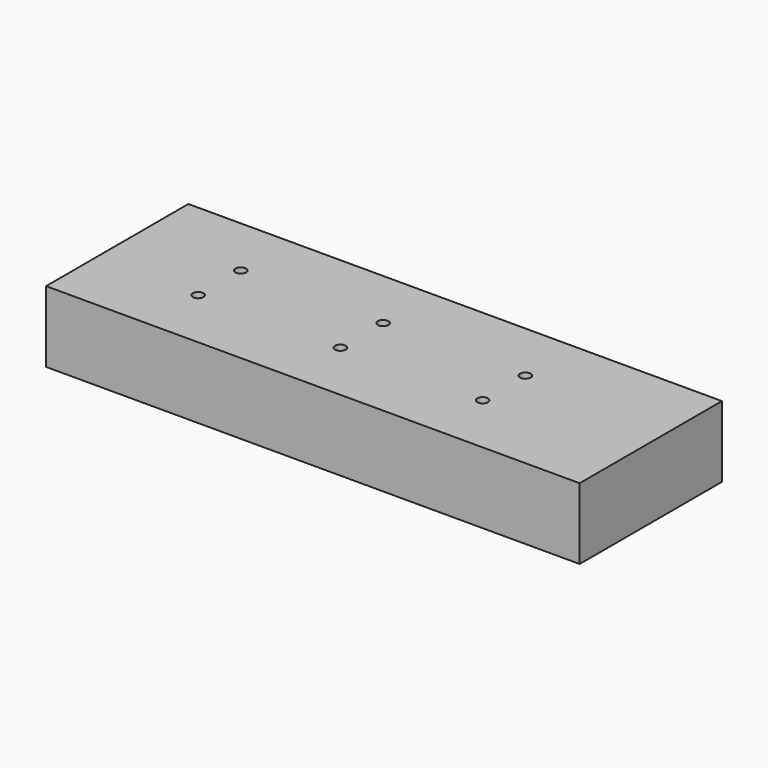
from build123d import *

# Parameters (mm, degrees)
F0_W     = 76.2
F0_H     = 25.4
F1_DEPTH = 10.16
F2_R     = 6.35
F3_DEPTH = 3.81


# Not quite as in the source:
# - a pattern or mirror of a feature is missing from the dataset's text; its kind, count and spacing are read off the source's solid


with BuildPart() as f1:
    # F0 (on Top) → F1 (new body)
    with BuildSketch(Plane.XY):
        Rectangle(F0_W, F0_H)
    extrude(amount=F1_DEPTH)

    # F2 (on face) → F3 (cut)
    with BuildSketch(Plane(origin=(0, 0, 0), x_dir=(1, 0, 0), z_dir=(0, 0, -1))):
        with Locations((-23.495, 0)):
            Circle(F2_R)
        with Locations((-3.175, 0)):
            Circle(F2_R)
        with Locations((17.145, 0)):
            Circle(F2_R)
    extrude(amount=-F3_DEPTH, mode=Mode.SUBTRACT)

    # F5 (on offset) → F6 (revolve, cut)
    with BuildSketch(Plane.XZ.offset(3.81)):
        Polygon((-26.035, 3.81), (-23.495, 3.81), (-23.495, 10.4205608368), (-24.257, 10.4205608368), (-24.257, 4.4571390765), align=None)
    f6 = revolve(axis=Axis((-23.495, -3.81, 7.1152804184), (0, 0, -1)), mode=Mode.SUBTRACT)

    # F6_copies: F6 across plane
    add(f6.mirror(Plane.ZX), mode=Mode.SUBTRACT)

    # F7 (on offset) → F8 (revolve, cut)
    with BuildSketch(Plane.XZ.offset(3.81)):
        Polygon((-5.715, 3.81), (-3.175, 3.81), (-3.175, 10.4205607442), (-3.937, 10.4205607442), (-3.937, 4.4571389839), align=None)
    f8 = revolve(axis=Axis((-3.175, -3.81, 10.0472030926), (0, 0, 1)), mode=Mode.SUBTRACT)

    # F8_copies: F8 across plane
    add(f8.mirror(Plane.ZX), mode=Mode.SUBTRACT)

    # F9 (on offset) → F10 (revolve, cut)
    with BuildSketch(Plane.XZ.offset(3.81)):
        Polygon((14.605, 3.81), (17.145, 3.81), (17.145, 10.4205608368), (16.383, 10.4205608368), (16.383, 4.4571390765), align=None)
    f10 = revolve(axis=Axis((17.145, -3.81, 8.0366932552), (0, 0, 1)), mode=Mode.SUBTRACT)

    # F10_copies: F10 across plane
    add(f10.mirror(Plane.ZX), mode=Mode.SUBTRACT)


solid = f1.part
